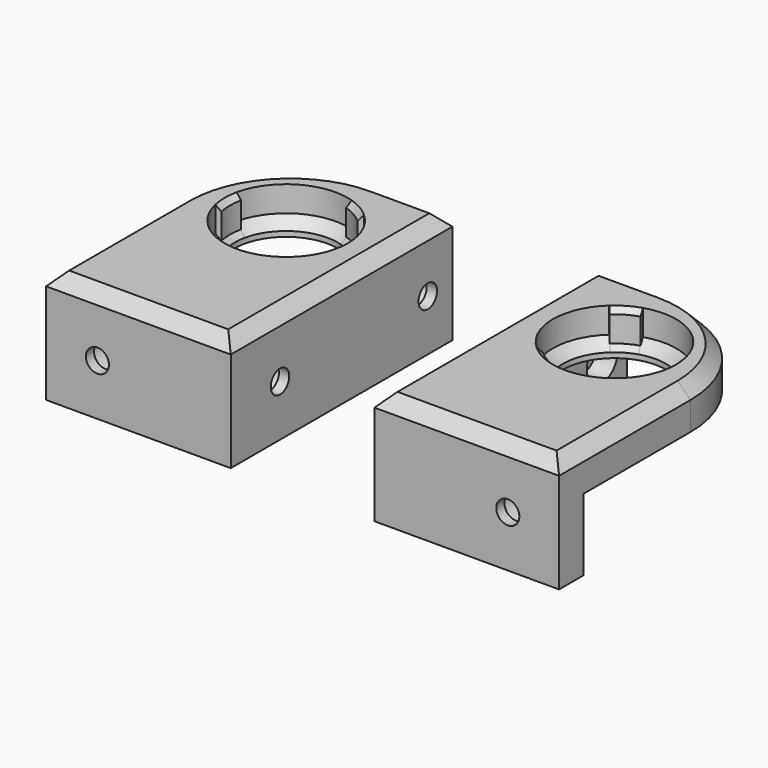
from build123d import *

# Parameters (mm, degrees)
F0_W      = 36
F0_H      = 54
F0_R      = 10
F1_DEPTH  = 8
F3_DEPTH  = 14
F4_R      = 2.25
F5_DEPTH  = 6.001
F6_R      = 3.75
F7_DEPTH  = 4
F8_R      = 2.25
F9_DEPTH  = 6.001
F10_R     = 3.75
F11_DEPTH = 4
F13_DEPTH = 7
F14_R     = 22
F15_SIZE  = 2.5
F16_SIZE  = 0.99999
F17_SIZE  = 1.9999


# Not quite as in the source:
# - a fillet or chamfer is up to 0.001 mm smaller than in the source, because OpenCascade refuses the exact size


with BuildPart() as f1:
    # F0 (on Top) → F1 (new body)
    with BuildSketch(Plane.XY):
        with Locations((18, 27)):
            Rectangle(F0_W, F0_H)
        with Locations((18, 36)):
            Circle(F0_R, mode=Mode.SUBTRACT)
    extrude(amount=F1_DEPTH)

    # F2 (on face) → F3 (join)
    with BuildSketch(Plane(origin=(0, 0, 0), x_dir=(1, 0, 0), z_dir=(0, 0, -1))):
        Polygon((36, 0), (0, 0), (0, -6), (30, -6), (30, -54), (36, -54), align=None)
    extrude(amount=F3_DEPTH)

    # F4 (on face) → F5 (cut, through all)
    with BuildSketch(Plane(origin=(0, 6, 0), x_dir=(-1, 0, 0), z_dir=(0, 1, 0))):
        with Locations((-10, -4)):
            Circle(F4_R)
    extrude(amount=-F5_DEPTH, mode=Mode.SUBTRACT)

    # F6 (on face) → F7 (cut)
    with BuildSketch(Plane(origin=(0, 6, 0), x_dir=(-1, 0, 0), z_dir=(0, 1, 0))):
        with Locations((-10, -4)):
            Circle(F6_R)
    extrude(amount=-F7_DEPTH, mode=Mode.SUBTRACT)

    # F8 (on face) → F9 (cut, through all)
    with BuildSketch(Plane(origin=(30, 0, 0), x_dir=(0, -1, 0), z_dir=(-1, 0, 0))):
        with Locations((-48, -4)):
            Circle(F8_R)
        with Locations((-12, -4)):
            Circle(F8_R)
    extrude(amount=-F9_DEPTH, mode=Mode.SUBTRACT)

    # F10 (on face) → F11 (cut)
    with BuildSketch(Plane(origin=(30, 0, 0), x_dir=(0, -1, 0), z_dir=(-1, 0, 0))):
        with Locations((-48, -4)):
            Circle(F10_R)
        with Locations((-12, -4)):
            Circle(F10_R)
    extrude(amount=-F11_DEPTH, mode=Mode.SUBTRACT)

    # F12 (on face) → F13 (cut)
    with BuildSketch(Plane.XY.offset(8)):
        with BuildLine():
            Line((21.3077637945, 46.4908864582), (21.6084695941, 47.444603409))
            ThreePointArc((21.6084695941, 47.444603409), (12, 46.3923048454), (6.2844479146, 38.5972753673))
            Line((6.2844479146, 38.5972753673), (7.2607439217, 38.3808357533))
            ThreePointArc((7.2607439217, 38.3808357533), (7, 36), (7.2607439217, 33.6191642467))
            Line((7.2607439217, 33.6191642467), (6.2844479146, 33.4027246327))
            ThreePointArc((6.2844479146, 33.4027246327), (12, 25.6076951546), (21.6084695941, 24.555396591))
            Line((21.6084695941, 24.555396591), (21.3077637945, 25.5091135418))
            ThreePointArc((21.3077637945, 25.5091135418), (23.5, 26.4737205584), (25.4314922838, 27.8899492951))
            Line((25.4314922838, 27.8899492951), (26.1070824914, 27.1526719583))
            ThreePointArc((26.1070824914, 27.1526719583), (30, 36), (26.1070824914, 44.8473280417))
            Line((26.1070824914, 44.8473280417), (25.4314922838, 44.1100507049))
            ThreePointArc((25.4314922838, 44.1100507049), (23.5, 45.5262794416), (21.3077637945, 46.4908864582))
        make_face()
    extrude(amount=-F13_DEPTH, mode=Mode.SUBTRACT)

    # F14
    f14_edges = [f1.edges().sort_by_distance(p)[0] for p in [
        (0, 54, 4),
    ]]
    fillet(f14_edges, radius=F14_R)

    # F15
    f15_edges = [f1.edges().sort_by_distance(p)[0] for p in [
        (36, 27, 8),
        (18, 0, 8),
        (29, 54, 8),
        (0, 16, 8),
    ]]
    chamfer(f15_edges, length=F15_SIZE)

    # F16 (size 1 in the source; OpenCascade refuses exactly that, so slightly less here)
    f16_edges = [f1.edges().sort_by_distance(p)[0] for p in [
        (23.5, 26.473721, 1),
        (7, 36, 1),
        (23.5, 45.526279, 1),
        (7, 36, 8),
        (23.5, 45.526279, 8),
        (23.5, 26.473721, 8),
    ]]
    chamfer(f16_edges, length=F16_SIZE)

    # F17 (size 2 in the source; OpenCascade refuses exactly that, so slightly less here)
    f17_edges = [f1.edges().sort_by_distance(p)[0] for p in [
        (12, 25.607695, 1),
        (30, 36, 1),
        (12, 46.392305, 1),
    ]]
    chamfer(f17_edges, length=F17_SIZE)


with BuildPart() as f19_1:
    # F19: instance of F1
    add(f1.part.mirror(Plane.YZ.offset(50)))


solid = Compound([f1.part, f19_1.part])
